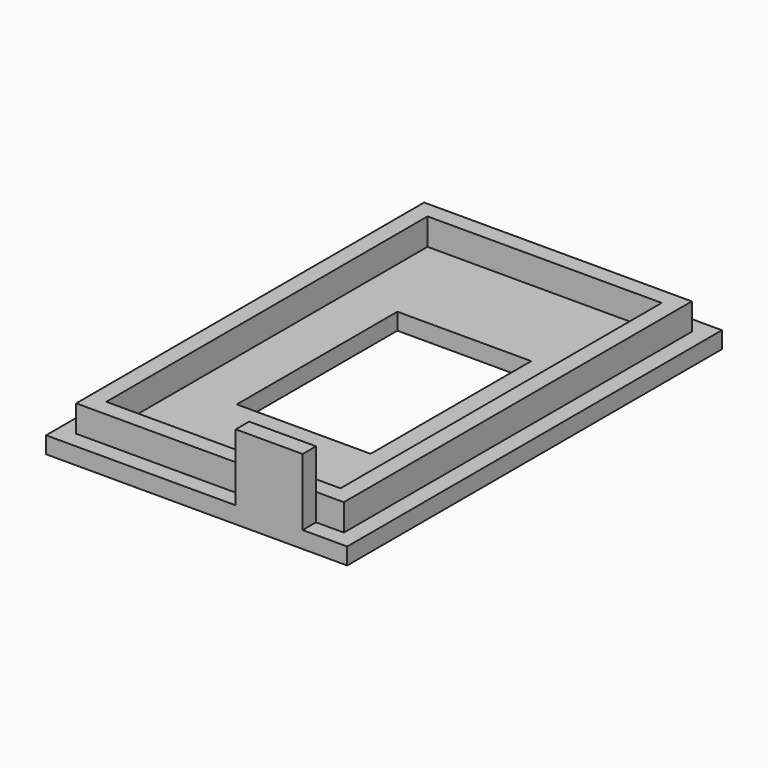
from build123d import *

# Parameters (mm, degrees)
F0_W        = 57.15
F0_H        = 88.9
F1_DEPTH    = 3.175
F2_W        = 50.8
F2_H        = 82.55
F3_DEPTH    = 5.08
F4_T        = 3.175
F4_T3_DEPTH = 57.15
F4_T5_DEPTH = 88.9
F5_W        = 25.4
F5_H        = 38.1
F6_DEPTH    = 25.4
F7_W        = 12.7
F7_H        = 7.62
F7_H_2      = 5.08
F8_DEPTH    = 3.175


# Not quite as in the source:
# - a shell that OpenCascade refuses in one call is made with other operations: the cavity is built on its own and cut out


with BuildPart() as f1:
    # F0 (on Top) → F1 (new body)
    with BuildSketch(Plane.XY):
        Rectangle(F0_W, F0_H)
    extrude(amount=F1_DEPTH)

    # F2 (on face) → F3 (join)
    with BuildSketch(Plane.XY.offset(3.175)):
        Rectangle(F2_W, F2_H)
    extrude(amount=F3_DEPTH)

    # F4: shell of thickness 3.175, made by hand


with BuildPart() as f4_core1:
    # F4_t2: copy of F1
    add(f1.part)

    # the walls: a layer under each face that stays
    f4_faces = [f4_core1.faces().sort_by_distance(p)[0] for p in [
        (0, 44.45, 1.5875),
        (28.575, 0, 1.5875),
        (-28.575, 0, 1.5875),
        (0, 0, 0),
        (-26.67, -41.4866666667, 3.175),
        (0, -44.45, 1.5875),
        (0, 41.275, 5.715),
        (-25.4, 0, 5.715),
        (0, -41.275, 5.715),
        (25.4, 0, 5.715),
    ]]
    thicken(f4_faces, amount=-F4_T, mode=Mode.SUBTRACT)

    # F4_s4 → F4_t3 (cut)
    with BuildSketch(Plane.YZ.offset(-28.575)):
        Polygon((41.30675, 3.20675), (41.275, 0), (38.1, 0), (38.1, 3.175), align=None)
        Polygon((-41.30675, 3.20675), (-41.275, 0), (-38.1, 0), (-38.1, 3.175), align=None)
    extrude(amount=F4_T3_DEPTH, mode=Mode.SUBTRACT)

    # F4_s6 → F4_t5 (cut)
    with BuildSketch(Plane.XZ.offset(-44.45)):
        Polygon((-25.43175, 3.20675), (-25.4, 0), (-22.225, 0), (-22.225, 3.175), align=None)
        Polygon((25.43175, 3.20675), (25.4, 0), (22.225, 0), (22.225, 3.175), align=None)
    extrude(amount=F4_T5_DEPTH, mode=Mode.SUBTRACT)


with BuildPart() as f1_1:
    add(f1.part)

    # what is left inside the walls is the cavity
    f4_cavity = [f4_core1.part.solids().sort_by_distance(p)[0] for p in [
        (0, -12.7, 3.20675),
    ]]
    add(f4_cavity, mode=Mode.SUBTRACT)

    # F5 (on face) → F6 (cut)
    with BuildSketch(Plane.XY.offset(3.175)):
        Rectangle(F5_W, F5_H)
    extrude(amount=-F6_DEPTH, mode=Mode.SUBTRACT)

    # F7 (on face) → F8 (join)
    with BuildSketch(Plane.XZ.offset(41.275)):
        with Locations((13.7679782532, 12.065)):
            Rectangle(F7_W, F7_H)
        with Locations((13.7679782532, 5.715)):
            Rectangle(F7_W, F7_H_2)
    extrude(amount=F8_DEPTH)


solid = f1_1.part
